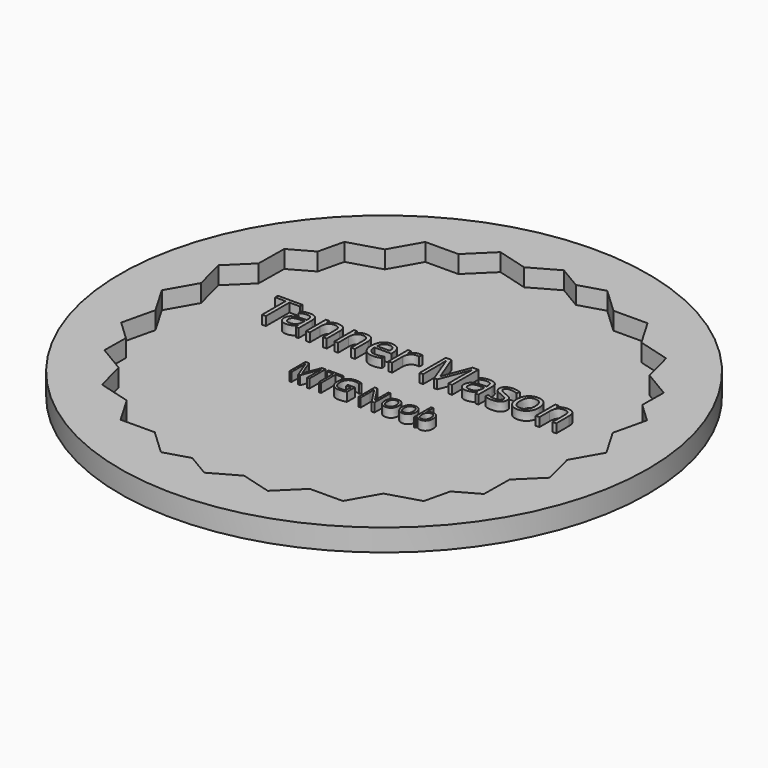
from build123d import *

# Parameters (mm, degrees)
F0_R           = 38.1
F1_DEPTH       = 3.175
F3_DEPTH       = 2.54
F4_TEXT_SIZE   = 6.630153588
F4_TEXT_SIZE_2 = 4.0896254682
F5_DEPTH       = 1.27


# Not quite as in the source:
# - Text() gives the source's letters only with a copy of the font that has no kerning and outlines rounded to 1/6400 em; it was checked with that copy


with BuildPart() as f1:
    # F0 (on Top) → F1 (new body)
    with BuildSketch(Plane.XY):
        Circle(F0_R)
    extrude(amount=F1_DEPTH)

    # F2 (on face) → F3 (cut)
    with BuildSketch(Plane.XY.offset(3.175)):
        Polygon((-16.7539807155, -22.2307116947), (-20.2813434379, -20.1346489786), (-18.2313309667, -23.6422477825), (-14.0041852642, -24.8207506786), align=None)
        Polygon((-15.8280923204, -27.7542213045), (-10.9174468457, -27.7281570579), (-14.0041852642, -24.8207506786), (-18.2313309667, -23.6422477825), align=None)
        Polygon((-7.5328270782, -27.7101925021), (-3.7128362491, -27.6899171262), (-10.9733600143, -25.6657265999), align=None)
        Polygon((0.2854385279, -28.8046121795), (-3.7128362491, -27.6899171262), (-7.5328270782, -27.7101925021), (-3.6848346955, -29.9967827964), align=None)
        Polygon((3.5707460553, -29.7205362351), (7.2964457928, -27.6314831294), (4.1364409877, -27.6482554956), (0.2854385279, -28.8046121795), align=None)
        Polygon((11.3591216989, -27.6099196532), (7.2964457928, -27.6314831294), (3.5707460553, -29.7205362351), (7.9575307916, -30.9435455373), align=None)
        Polygon((14.4933079966, -24.5383555374), (10.875370714, -25.6247287615), (7.2964457928, -27.6314831294), (11.3591216989, -27.6099196532), align=None)
        Polygon((16.1218145518, -27.5846406951), (18.5545649894, -23.3188648418), (14.4933079966, -24.5383555374), (11.3591216989, -27.6099196532), align=None)
        Polygon((21.8758711357, 17.4063907244), (20.2813434379, 20.1346489786), (16.7539807155, 22.2307116947), align=None)
        Polygon((20.2313171115, -20.3787158631), (22.1237535355, -17.0603690749), (16.7404912349, -22.3360718372), align=None)
        Polygon((25.0882451575, -14.1551090734), (22.1237535355, -17.0603690749), (20.2313171115, -20.3787158631), (24.1355585858, -18.1895518532), align=None)
        Polygon((27.5241124213, -11.7679113232), (27.5777892307, -7.4968341508), (26.0123121234, -10.2418647712), (25.0882451575, -14.1551090734), align=None)
        Polygon((29.5904526656, -3.9676718707), (27.5777892307, -7.4968341508), (27.5241124213, -11.7679113232), (30.7766619143, -8.5803489518), align=None)
        Polygon((28.4974932607, 0.2823951412), (27.6293514295, -3.3940170668), (27.5777892307, -7.4968341508), (29.5904526656, -3.9676718707), align=None)
        Polygon((31.9499068721, 0.1695806094), (29.4720118351, 4.4092922161), (28.4974932607, 0.2823951412), (29.5904526656, -3.9676718707), align=None)
        Polygon((27.7641441897, 7.331476639), (25.8365897845, 10.6295480513), (27.7138512493, 3.3296547627), align=None)
        Polygon((24.8028066296, 14.6495031061), (25.8365897845, 10.6295480513), (27.7641441897, 7.331476639), (27.8203932812, 11.8072309432), align=None)
        Polygon((23.953366366, 17.9526249119), (20.2813434379, 20.1346489786), (21.8758711357, 17.4063907244), (24.8028066296, 14.6495031061), align=None)
        Polygon((22.8191311227, 22.3631965856), (18.2313309667, 23.6422477825), (20.2813434379, 20.1346489786), (23.953366366, 17.9526249119), align=None)
        Polygon((20.2813434379, 20.1346489786), (18.2313309667, 23.6422477825), (14.0041852642, 24.8207506786), (16.7539807155, 22.2307116947), align=None)
        Polygon((18.2313309667, 23.6422477825), (15.8280923204, 27.7542213045), (10.9174468457, 27.7281570579), (14.0041852642, 24.8207506786), align=None)
        Polygon((3.7128362491, 27.6899171262), (7.5328270782, 27.7101925021), (3.6848346955, 29.9967827964), (-0.2854385279, 28.8046121795), align=None)
        Polygon((-7.2964457928, 27.6314831294), (-4.1364409877, 27.6482554956), (-0.2854385279, 28.8046121795), (-3.5707460553, 29.7205362351), align=None)
        Polygon((10.9733600143, 25.6657265999), (7.5328270782, 27.7101925021), (3.7128362491, 27.6899171262), align=None)
        Polygon((-10.875370714, 25.6247287615), (-7.2964457928, 27.6314831294), (-11.3591216989, 27.6099196532), (-14.4933079966, 24.5383555374), align=None)
        Polygon((-11.3591216989, 27.6099196532), (-7.2964457928, 27.6314831294), (-3.5707460553, 29.7205362351), (-7.9575307916, 30.9435455373), align=None)
        Polygon((-14.4933079966, 24.5383555374), (-11.3591216989, 27.6099196532), (-16.1218145518, 27.5846406951), (-18.5545649894, 23.3188648418), align=None)
        Polygon((-22.1237535355, 17.0603690749), (-16.7404912349, 22.3360718372), (-20.2313171115, 20.3787158631), align=None)
        Polygon((-22.1237535355, 17.0603690749), (-20.2313171115, 20.3787158631), (-24.1355585858, 18.1895518532), (-25.0882451575, 14.1551090734), align=None)
        Polygon((-27.5777892307, 7.4968341508), (-26.0123121234, 10.2418647712), (-25.0882451575, 14.1551090734), (-27.5241124213, 11.7679113232), align=None)
        Polygon((-29.5904526656, 3.9676718707), (-27.5777892307, 7.4968341508), (-27.5241124213, 11.7679113232), (-30.7766619143, 8.5803489518), align=None)
        Polygon((-27.6293514295, 3.3940170668), (-27.5777892307, 7.4968341508), (-29.5904526656, 3.9676718707), (-28.4974932607, -0.2823951412), align=None)
        Polygon((-28.4974932607, -0.2823951412), (-29.5904526656, 3.9676718707), (-31.9499068721, -0.1695806094), (-29.4720118351, -4.4092922161), align=None)
        Polygon((-25.8365897845, -10.6295480513), (-27.7138512493, -3.3296547627), (-27.7641441897, -7.331476639), align=None)
        Polygon((-20.2813434379, -20.1346489786), (-21.8758711357, -17.4063907244), (-24.8028066296, -14.6495031061), (-23.953366366, -17.9526249119), align=None)
        Polygon((-25.8365897845, -10.6295480513), (-27.7641441897, -7.331476639), (-27.8203932812, -11.8072309432), (-24.8028066296, -14.6495031061), align=None)
        Polygon((-24.8028066296, -14.6495031061), (-27.8203932812, -11.8072309432), (-27.8683882635, -15.6262037078), (-23.953366366, -17.9526249119), align=None)
        Polygon((-27.8203932812, -11.8072309432), (-27.7641441897, -7.331476639), (-29.4720118351, -4.4092922161), (-30.6005813396, -9.1885650892), align=None)
        Polygon((-27.7641441897, -7.331476639), (-27.7138512493, -3.3296547627), (-28.4974932607, -0.2823951412), (-29.4720118351, -4.4092922161), align=None)
        Polygon((-27.7138512493, -3.3296547627), (-27.6293514295, 3.3940170668), (-28.4974932607, -0.2823951412), align=None)
        Polygon((-27.6293514295, 3.3940170668), (-26.0123121234, 10.2418647712), (-27.5777892307, 7.4968341508), align=None)
        Polygon((-26.0123121234, 10.2418647712), (-22.1237535355, 17.0603690749), (-25.0882451575, 14.1551090734), align=None)
        Polygon((-25.0882451575, 14.1551090734), (-24.1355585858, 18.1895518532), (-27.4668835074, 16.3216303448), (-27.5241124213, 11.7679113232), align=None)
        Polygon((-24.1355585858, 18.1895518532), (-20.2313171115, 20.3787158631), (-18.5545649894, 23.3188648418), (-23.2578214614, 21.9065982661), align=None)
        Polygon((7.5328270782, 27.7101925021), (10.9174468457, 27.7281570579), (7.3427598783, 31.0951633553), (3.6848346955, 29.9967827964), align=None)
        Polygon((-0.2854385279, 28.8046121795), (3.6848346955, 29.9967827964), (0.4015047561, 31.9478340526), (-3.5707460553, 29.7205362351), align=None)
        Polygon((-4.1364409877, 27.6482554956), (3.7128362491, 27.6899171262), (-0.2854385279, 28.8046121795), align=None)
        Polygon((-10.875370714, 25.6247287615), (-4.1364409877, 27.6482554956), (-7.2964457928, 27.6314831294), align=None)
        Polygon((-20.2313171115, 20.3787158631), (-16.7404912349, 22.3360718372), (-14.4933079966, 24.5383555374), (-18.5545649894, 23.3188648418), align=None)
        Polygon((27.8203932812, 11.8072309432), (27.7641441897, 7.331476639), (29.4720118351, 4.4092922161), (30.6005813396, 9.1885650892), align=None)
        Polygon((27.8683882635, 15.6262037078), (23.953366366, 17.9526249119), (24.8028066296, 14.6495031061), (27.8203932812, 11.8072309432), align=None)
        Polygon((29.4720118351, 4.4092922161), (27.7641441897, 7.331476639), (27.7138512493, 3.3296547627), (28.4974932607, 0.2823951412), align=None)
        Polygon((27.4668835074, -16.3216303448), (27.5241124213, -11.7679113232), (25.0882451575, -14.1551090734), (24.1355585858, -18.1895518532), align=None)
        Polygon((24.1355585858, -18.1895518532), (20.2313171115, -20.3787158631), (18.5545649894, -23.3188648418), (23.2578214614, -21.9065982661), align=None)
        Polygon((18.5545649894, -23.3188648418), (20.2313171115, -20.3787158631), (16.7404912349, -22.3360718372), (14.4933079966, -24.5383555374), align=None)
        Polygon((-0.4015047561, -31.9478340526), (3.5707460553, -29.7205362351), (0.2854385279, -28.8046121795), (-3.6848346955, -29.9967827964), align=None)
        Polygon((-3.6848346955, -29.9967827964), (-7.5328270782, -27.7101925021), (-10.9174468457, -27.7281570579), (-7.3427598783, -31.0951633553), align=None)
        Polygon((-10.9174468457, -27.7281570579), (-7.5328270782, -27.7101925021), (-10.9733600143, -25.6657265999), (-14.0041852642, -24.8207506786), align=None)
        Polygon((14.0041852642, 24.8207506786), (10.9174468457, 27.7281570579), (7.5328270782, 27.7101925021), (10.9733600143, 25.6657265999), align=None)
        Polygon((25.8365897845, 10.6295480513), (21.8758711357, 17.4063907244), (16.7539807155, 22.2307116947), (10.9733600143, 25.6657265999), (3.7128362491, 27.6899171262), (-4.1364409877, 27.6482554956), (-10.875370714, 25.6247287615), (-16.7404912349, 22.3360718372), (-22.1237535355, 17.0603690749), (-26.0123121234, 10.2418647712), (-27.6293514295, 3.3940170668), (-27.7138512493, -3.3296547627), (-25.8365897845, -10.6295480513), (-21.8758711357, -17.4063907244), (-16.7539807155, -22.2307116947), (-10.9733600143, -25.6657265999), (-3.7128362491, -27.6899171262), (4.1364409877, -27.6482554956), (10.875370714, -25.6247287615), (16.7404912349, -22.3360718372), (22.1237535355, -17.0603690749), (26.0123121234, -10.2418647712), (27.6293514295, -3.3940170668), (27.7138512493, 3.3296547627), align=None)
        Polygon((27.5777892307, -7.4968341508), (27.6293514295, -3.3940170668), (26.0123121234, -10.2418647712), align=None)
        Polygon((25.0882451575, -14.1551090734), (26.0123121234, -10.2418647712), (22.1237535355, -17.0603690749), align=None)
        Polygon((7.2964457928, -27.6314831294), (10.875370714, -25.6247287615), (4.1364409877, -27.6482554956), align=None)
        Polygon((14.4933079966, -24.5383555374), (16.7404912349, -22.3360718372), (10.875370714, -25.6247287615), align=None)
        Polygon((0.2854385279, -28.8046121795), (4.1364409877, -27.6482554956), (-3.7128362491, -27.6899171262), align=None)
        Polygon((-14.0041852642, -24.8207506786), (-10.9733600143, -25.6657265999), (-16.7539807155, -22.2307116947), align=None)
        Polygon((-18.2313309667, -23.6422477825), (-20.2813434379, -20.1346489786), (-23.953366366, -17.9526249119), (-22.8191311227, -22.3631965856), align=None)
        Polygon((-21.8758711357, -17.4063907244), (-25.8365897845, -10.6295480513), (-24.8028066296, -14.6495031061), align=None)
        Polygon((-16.7539807155, -22.2307116947), (-21.8758711357, -17.4063907244), (-20.2813434379, -20.1346489786), align=None)
        Polygon((16.7539807155, 22.2307116947), (14.0041852642, 24.8207506786), (10.9733600143, 25.6657265999), align=None)
        Polygon((-16.7404912349, 22.3360718372), (-10.875370714, 25.6247287615), (-14.4933079966, 24.5383555374), align=None)
        Polygon((24.8028066296, 14.6495031061), (21.8758711357, 17.4063907244), (25.8365897845, 10.6295480513), align=None)
        Polygon((28.4974932607, 0.2823951412), (27.7138512493, 3.3296547627), (27.6293514295, -3.3940170668), align=None)
    extrude(amount=-F3_DEPTH, mode=Mode.SUBTRACT)

    # F4 (on face) → F5 (join)
    with BuildSketch(Plane.XY.offset(0.635)):
        with Locations((-22.475631367, 4.1343280102)):
            Text('Tanner Mason', F4_TEXT_SIZE, font='Open Sans', text_align=(TextAlign.LEFT, TextAlign.BOTTOM))
        with Locations((-10.3058563545, -4.7214021906)):
            Text('MTG Noob', F4_TEXT_SIZE_2, font='Open Sans', text_align=(TextAlign.LEFT, TextAlign.BOTTOM))
    extrude(amount=F5_DEPTH)


solid = f1.part
